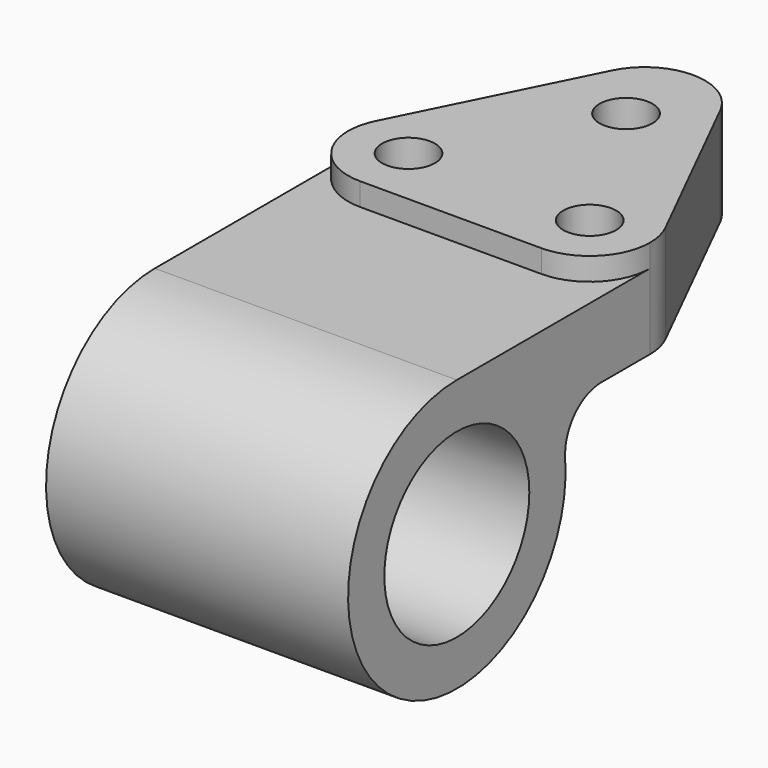
from build123d import *

# Parameters (mm, degrees)
F0_R     = 19.05
F1_DEPTH = 31.75
F3_DEPTH = 43.06758
F4_DEPTH = 25.4
F5_DEPTH = 4.7752
F6_DEPTH = 4.7752
F2_R     = 5.5626
F7_DEPTH = 61.9262
F8_DEPTH = 4.7625


with BuildPart() as f1:
    # F0 (on Right) → F1 (new body, symmetric)
    with BuildSketch(Plane.YZ):
        with BuildLine():
            Line((38.1, 28.575), (0, 28.575))
            ThreePointArc((0, 28.575), (-27.3235693319, -8.3638020041), (15.9950252975, -23.6788891364))
            ThreePointArc((15.9950252975, -23.6788891364), (25.7719232537, -12.3425522809), (28.4756083945, 2.38125))
            ThreePointArc((28.4756083945, 2.38125), (30.9572676717, 9.6234554837), (37.9674778593, 12.7))
            Line((37.9674778593, 12.7), (69.85, 12.7))
            Line((69.85, 12.7), (101.7325221407, 12.7))
            Line((101.7325221407, 12.7), (101.7325221407, 33.3502))
            Line((101.7325221407, 33.3502), (38.1, 33.3502))
            Line((38.1, 33.3502), (38.1, 28.575))
        make_face()
        Circle(F0_R, mode=Mode.SUBTRACT)
    extrude(amount=F1_DEPTH, both=True)

    # F2 (on face) → F3 (cut)
    with BuildSketch(Plane.XY.offset(33.3502)):
        with BuildLine():
            ThreePointArc((30.4170945511, 56.4638468789), (31.4122833813, 53.7092867856), (31.75, 50.8))
            Line((31.75, 50.8), (31.75, 101.7325221407))
            Line((31.75, 101.7325221407), (-1.274e-07, 101.7325221407))
            ThreePointArc((-1.274e-07, 101.7325221407), (6.6842779412, 99.8311529985), (11.3670945511, 94.6963690195))
            Line((11.3670945511, 94.6963690195), (30.4170945511, 56.4638468789))
        make_face()
    extrude(amount=-F3_DEPTH, mode=Mode.SUBTRACT)

    # F2 (on face) → F4 (cut)
    with BuildSketch(Plane.XY.offset(33.3502)):
        with BuildLine():
            Line((-31.75, 101.7325221407), (-31.75, 50.8))
            ThreePointArc((-31.75, 50.8), (-31.4122833813, 53.7092867856), (-30.4170945511, 56.4638468789))
            Line((-30.4170945511, 56.4638468789), (-11.3670945511, 94.6963690195))
            ThreePointArc((-11.3670945511, 94.6963690195), (-6.6842780495, 99.8311529315), (-1.274e-07, 101.7325221407))
            Line((-1.274e-07, 101.7325221407), (-31.75, 101.7325221407))
        make_face()
    extrude(amount=-F4_DEPTH, mode=Mode.SUBTRACT)

    # F2 (on face) → F5 (cut)
    with BuildSketch(Plane.XY.offset(33.3502)):
        with BuildLine():
            Line((-31.75, 38.1), (-19.05, 38.1))
            ThreePointArc((-19.05, 38.1), (-28.0302561211, 41.8197438789), (-31.75, 50.8))
            Line((-31.75, 50.8), (-31.75, 38.1))
        make_face()
    extrude(amount=-F5_DEPTH, mode=Mode.SUBTRACT)

    # F2 (on face) → F6 (cut)
    with BuildSketch(Plane.XY.offset(33.3502)):
        with BuildLine():
            ThreePointArc((31.75, 50.8), (28.0302561211, 41.8197438789), (19.05, 38.1))
            Line((19.05, 38.1), (31.75, 38.1))
            Line((31.75, 38.1), (31.75, 50.8))
        make_face()
    extrude(amount=-F6_DEPTH, mode=Mode.SUBTRACT)

    # F2 (on face) → F7 (cut, through all)
    with BuildSketch(Plane.XY.offset(33.3502)):
        with Locations((-19.05, 50.8)):
            Circle(F2_R)
        with Locations((0, 84.1502)):
            Circle(F2_R)
        with Locations((19.05, 50.8)):
            Circle(F2_R)
    extrude(amount=-F7_DEPTH, mode=Mode.SUBTRACT)

    # F0 (on Right) → F8 (join, symmetric)
    with BuildSketch(Plane.YZ):
        with BuildLine():
            ThreePointArc((28.4756083945, 2.38125), (25.7719232537, -12.3425522809), (15.9950252975, -23.6788891364))
            Line((15.9950252975, -23.6788891364), (69.85, 12.7))
            Line((69.85, 12.7), (37.9674778593, 12.7))
            ThreePointArc((37.9674778593, 12.7), (30.9572676717, 9.6234554837), (28.4756083945, 2.38125))
        make_face()
    extrude(amount=F8_DEPTH, both=True)


solid = f1.part
